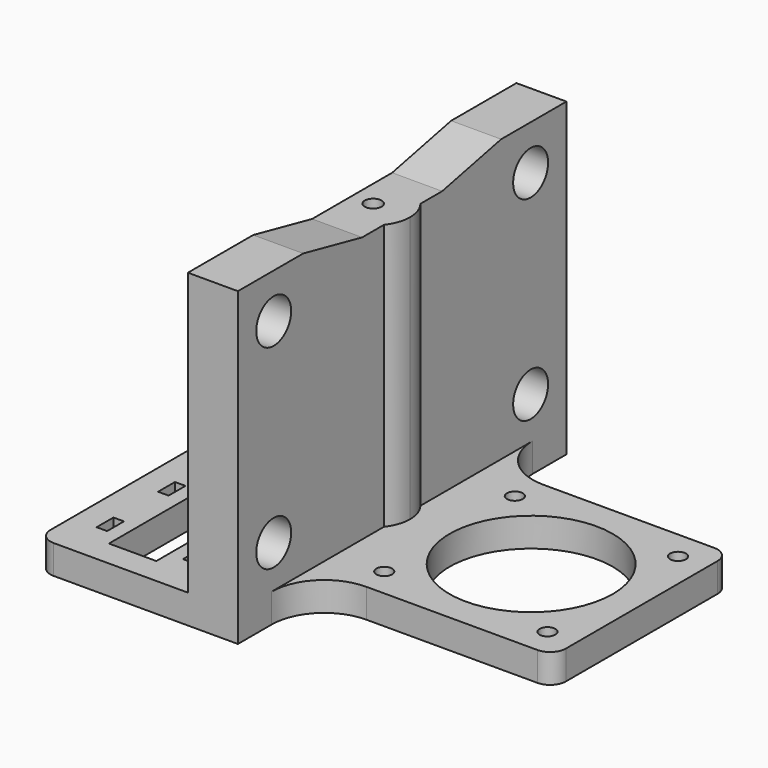
from build123d import *

# Parameters (mm, degrees)
F0_W         = 51
F0_H         = 42
F0_R         = 1.5
F0_R_2       = 15.5
F4_DEPTH     = 5.5
F1_W         = 32.5
F1_H         = 39
F1_W_2       = 2
F1_H_2       = 4
F1_W_3       = 9
F1_H_3       = 24.5
F5_DEPTH     = 5.5
F6_DEPTH     = 59
F3_W         = 27.5
F3_H         = 4
F7_DEPTH     = 56
F8_R         = 4.15
F9_DEPTH     = 6
F10_DEPTH    = 40
F11_DEPTH    = 153
F12_R        = 10
F13_R        = 3
F15_DEPTH    = 10.56991
F16_T4_DEPTH = 265.6917724847
F16_T9_DEPTH = 265.6917724847


# Not quite as in the source:
# - a fillet or chamfer that OpenCascade refuses, or shapes differently, is made with other operations: its cross-section is extruded or revolved along the edge and cut away or added
# - an extrude ends at something that could not be found from the text; its depth is read off the source's solid
# - a pattern or mirror of a feature is missing from the dataset's text; its kind, count and spacing are read off the source's solid


with BuildPart() as f4:
    # F0 (on Top) → F4 (new body)
    with BuildSketch(Plane.XY):
        with Locations((25.5, 0)):
            Rectangle(F0_W, F0_H)
        with Locations((14.5, -15.5)):
            Circle(F0_R, mode=Mode.SUBTRACT)
        with Locations((45.5, -15.5)):
            Circle(F0_R, mode=Mode.SUBTRACT)
        with Locations((14.5, 15.5)):
            Circle(F0_R, mode=Mode.SUBTRACT)
        with Locations((30, 0)):
            Circle(F0_R_2, mode=Mode.SUBTRACT)
        with Locations((45.5, 15.5)):
            Circle(F0_R, mode=Mode.SUBTRACT)
    extrude(amount=F4_DEPTH)

    # F1 (on Top) → F5 (join, through all)
    with BuildSketch(Plane.XY):
        with Locations((-16.25, -19.5)):
            Rectangle(F1_W, F1_H)
        with Locations((-26.7, -29.05)):
            Rectangle(F1_W_2, F1_H_2, mode=Mode.SUBTRACT)
        with Locations((-18.5, -21.75)):
            Rectangle(F1_W_3, F1_H_3, mode=Mode.SUBTRACT)
        with Locations((-10.3, -29.05)):
            Rectangle(F1_W_2, F1_H_2, mode=Mode.SUBTRACT)
        with Locations((-26.7, -14.45)):
            Rectangle(F1_W_2, F1_H_2, mode=Mode.SUBTRACT)
        with Locations((-10.3, -14.45)):
            Rectangle(F1_W_2, F1_H_2, mode=Mode.SUBTRACT)
    f5 = extrude(amount=F5_DEPTH)

    # F5_copies: F5 across plane
    add(f5.mirror(Plane.ZX))

    # F2 (on Top) → F6 (join)
    with BuildSketch(Plane.XY):
        with BuildLine():
            ThreePointArc((5.5, -4.3301270189), (1.0308525773, -6.9236798716), (-4, -5.7445626465))
            Line((-4, -5.7445626465), (-4, -39))
            Line((-4, -39), (5.5, -39))
            Line((5.5, -39), (5.5, -4.3301270189))
        make_face()
        with BuildLine():
            Line((-4, 0), (-4, -5.7445626465))
            ThreePointArc((-4, -5.7445626465), (1.0308525773, -6.9236798716), (5.5, -4.3301270189))
            Line((5.5, -4.3301270189), (5.5, 0))
            Line((5.5, 0), (4, 0))
            ThreePointArc((4, 0), (0, -4), (-4, 0))
        make_face()
        with BuildLine():
            ThreePointArc((5.5, -4.3301270189), (6.6143782777, -2.2912878475), (7, 0))
            ThreePointArc((7, 0), (-3.2403703492, 6.204836823), (-4, -5.7445626465))
            Line((-4, -5.7445626465), (-4, 0))
            ThreePointArc((-4, 0), (0, 4), (4, 0))
            Line((4, 0), (5.5, 0))
            Line((5.5, 0), (5.5, -4.3301270189))
        make_face()
        with BuildLine():
            Line((-1.6, 0), (-4, 0))
            ThreePointArc((-4, 0), (0, -4), (4, 0))
            Line((4, 0), (1.6, 0))
            ThreePointArc((1.6, 0), (0, -1.6), (-1.6, 0))
        make_face()
        with BuildLine():
            ThreePointArc((4, 0), (0, 4), (-4, 0))
            Line((-4, 0), (-1.6, 0))
            ThreePointArc((-1.6, 0), (0, 1.6), (1.6, 0))
            Line((1.6, 0), (4, 0))
        make_face()
        with BuildLine():
            ThreePointArc((1.6, 0), (0, 1.6), (-1.6, 0))
            Line((-1.6, 0), (1.6, 0))
        make_face()
        with BuildLine():
            Line((1.6, 0), (-1.6, 0))
            ThreePointArc((-1.6, 0), (0, -1.6), (1.6, 0))
        make_face()
    f6 = extrude(amount=F6_DEPTH)

    # F6_copies: F6 across plane
    add(f6.mirror(Plane.ZX))

    # F3 (on Top) → F7 (join)
    with BuildSketch(Plane.XY):
        with Locations((-13.75, -7.5)):
            Rectangle(F3_W, F3_H)
    f7 = extrude(amount=F7_DEPTH)

    # F7_copies: F7 across plane
    add(f7.mirror(Plane.ZX.offset(-9e-06)))

    # F8 (on Right) → F9 (cut, symmetric)
    with BuildSketch(Plane.YZ):
        with Locations((30.5, 50.5481660366)):
            Circle(F8_R)
        with Locations((30.5, 13.5)):
            Circle(F8_R)
        with Locations((-30.5, 13.5)):
            Circle(F8_R)
        with Locations((-30.5, 50.5481660366)):
            Circle(F8_R)
    extrude(amount=F9_DEPTH, both=True, mode=Mode.SUBTRACT)

    # F2 (on Top) → F10 (cut)
    with BuildSketch(Plane.XY):
        with BuildLine():
            Line((-1.6, 0), (-4, 0))
            ThreePointArc((-4, 0), (0, -4), (4, 0))
            Line((4, 0), (1.6, 0))
            ThreePointArc((1.6, 0), (0, -1.6), (-1.6, 0))
        make_face()
        with BuildLine():
            ThreePointArc((4, 0), (0, 4), (-4, 0))
            Line((-4, 0), (-1.6, 0))
            ThreePointArc((-1.6, 0), (0, 1.6), (1.6, 0))
            Line((1.6, 0), (4, 0))
        make_face()
        with BuildLine():
            ThreePointArc((1.6, 0), (0, 1.6), (-1.6, 0))
            Line((-1.6, 0), (1.6, 0))
        make_face()
        with BuildLine():
            Line((1.6, 0), (-1.6, 0))
            ThreePointArc((-1.6, 0), (0, -1.6), (1.6, 0))
        make_face()
    extrude(amount=F10_DEPTH, mode=Mode.SUBTRACT)

    # F2 (on Top) → F11 (cut, through all)
    with BuildSketch(Plane.XY):
        with BuildLine():
            Line((1.6, 0), (-1.6, 0))
            ThreePointArc((-1.6, 0), (0, -1.6), (1.6, 0))
        make_face()
        with BuildLine():
            ThreePointArc((1.6, 0), (0, 1.6), (-1.6, 0))
            Line((-1.6, 0), (1.6, 0))
        make_face()
    extrude(amount=F11_DEPTH, mode=Mode.SUBTRACT)

    # F12
    f12_edges = [f4.edges().sort_by_distance(p)[0] for p in [
        (5.5, -21, 2.75),
        (5.5, 21, 2.75),
    ]]
    fillet(f12_edges, radius=F12_R)

    # F13
    f13_edges = [f4.edges().sort_by_distance(p)[0] for p in [
        (51, 21, 2.75),
        (51, -21, 2.75),
        (-32.5, -39, 2.75),
        (-32.5, 39, 2.75),
    ]]
    fillet(f13_edges, radius=F13_R)

    # F14 (on Right) → F15 (cut, symmetric)
    with BuildSketch(Plane.YZ):
        Polygon((23.5, 59), (-23.5, 59), (-9.5, 56), (9.5, 56), align=None)
    extrude(amount=F15_DEPTH, both=True, mode=Mode.SUBTRACT)

    # F16: chamfer of 23.5 x 50.5 on 2 edges, made by hand


with BuildPart() as f16_tool2:
    # F16_s3 → F16_t4 (new body)
    with BuildSketch(Plane.XZ.offset(-125.3458862424)):
        Polygon((-27.5, 5.5), (-4, 56), (-27.5, 56), align=None)
    extrude(amount=F16_T4_DEPTH)

    split(bisect_by=Plane.XY.offset(5.5), keep=Keep.TOP)


with BuildPart() as f4_1:
    add(f4.part)

    # F16_t1: cut F16_tool2
    add(f16_tool2.part, mode=Mode.SUBTRACT)


with BuildPart() as f16_tool7:
    # F16_s8 → F16_t9 (new body)
    with BuildSketch(Plane.XZ.offset(125.3459042424)):
        Polygon((-27.5, 5.5), (-4, 56), (-27.5, 56), align=None)
    extrude(amount=-F16_T9_DEPTH)

    split(bisect_by=Plane.XY.offset(5.5), keep=Keep.TOP)


with BuildPart() as f4_2:
    add(f4_1.part)

    # F16_t6: cut F16_tool7
    add(f16_tool7.part, mode=Mode.SUBTRACT)


solid = f4_2.part
